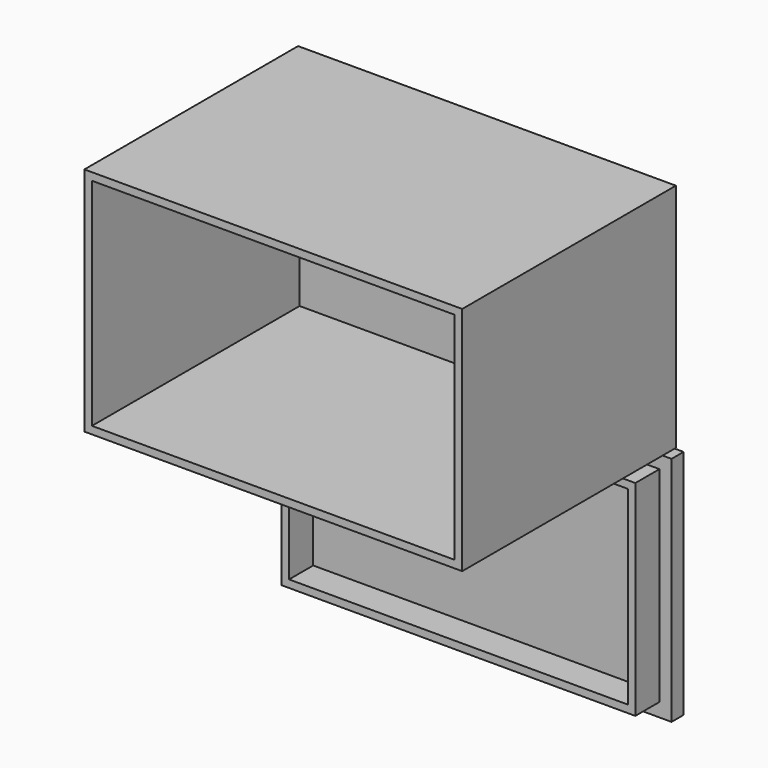
from build123d import *

# Parameters (mm, degrees)
F0_W        = 127.1928735077
F0_H        = 77.7173149399
F1_DEPTH    = 89.916
F2_T        = -2.54
F3_W        = 127.5507546961
F3_H        = 77.9658099636
F4_DEPTH    = 2.54
F5_W        = 119.1201396286
F5_H        = 69.0140379593
F6_DEPTH    = 10.16
F9_T        = 2.54
F9_T3_DEPTH = 124.2001396286
F9_T5_DEPTH = 74.0940379593
F8_W        = 127.5507546961
F8_H        = 77.9658099636
F8_W_2      = 46.9547603279
F8_H_2      = 47.2698919475
F8_W_3      = 21.6541066766
F8_H_3      = 15.249369666
F10_DEPTH   = 2.54


# Not quite as in the source:
# - a shell that OpenCascade refuses in one call is made with other operations: the cavity is built on its own and cut out


with BuildPart() as f1:
    # F0 (on Front) → F1 (new body)
    with BuildSketch(Plane.XZ):
        with Locations((-83.7561842054, 32.0948308799)):
            Rectangle(F0_W, F0_H)
    extrude(amount=F1_DEPTH)

    # F2
    f2_openings = [f1.faces().sort_by_distance(p)[0] for p in [
        (-83.756184, -89.916, 32.094831),
    ]]
    offset(amount=F2_T, openings=f2_openings)


with BuildPart() as f4:
    # F3 (on Front) → F4 (new body)
    with BuildSketch(Plane.XZ):
        with Locations((-83.3670627326, -47.7856700309)):
            Rectangle(F3_W, F3_H)
    extrude(amount=F4_DEPTH)

    # F5 (on face) → F6 (join)
    with BuildSketch(Plane.XZ.offset(2.54)):
        with Locations((-83.2092221826, -47.6696216501)):
            Rectangle(F5_W, F5_H)
    extrude(amount=F6_DEPTH)

    # F9: shell of thickness 2.54, made by hand


with BuildPart() as f9_core1:
    # F9_t2: copy of F4
    add(f4.part)

    # the walls: a layer under each face that stays
    f9_faces = [f9_core1.faces().sort_by_distance(p)[0] for p in [
        (-83.3670627326, -1.27, -8.802765049),
        (-19.5916853845, -1.27, -47.7856700309),
        (-147.1424400806, -1.27, -47.7856700309),
        (-83.3670627326, 0, -47.7856700309),
        (-142.8907482574, -2.54, -84.1697146806),
        (-83.3670627326, -1.27, -86.7685750127),
        (-83.2092221826, -7.62, -13.1626026705),
        (-142.769291997, -7.62, -47.6696216501),
        (-83.2092221826, -7.62, -82.1766406298),
        (-23.6491523683, -7.62, -47.6696216501),
    ]]
    thicken(f9_faces, amount=-F9_T, mode=Mode.SUBTRACT)

    # F9_s4 → F9_t3 (cut)
    with BuildSketch(Plane.YZ.offset(-145.309291997)):
        Polygon((-2.5654, -13.1372026705), (0, -13.1626026705), (0, -15.7026026705), (-2.54, -15.7026026705), align=None)
        Polygon((-2.5654, -82.2020406298), (0, -82.1766406298), (0, -79.6366406298), (-2.54, -79.6366406298), align=None)
    extrude(amount=F9_T3_DEPTH, mode=Mode.SUBTRACT)

    # F9_s6 → F9_t5 (cut)
    with BuildSketch(Plane.XY.offset(-84.7166406298)):
        Polygon((-142.794691997, -2.5654), (-142.769291997, 0), (-140.229291997, 0), (-140.229291997, -2.54), align=None)
        Polygon((-23.6237523683, -2.5654), (-23.6491523683, 0), (-26.1891523683, 0), (-26.1891523683, -2.54), align=None)
    extrude(amount=F9_T5_DEPTH, mode=Mode.SUBTRACT)


with BuildPart() as f4_1:
    add(f4.part)

    # what is left inside the walls is the cavity
    f9_cavity = [f9_core1.part.solids().sort_by_distance(p)[0] for p in [
        (-83.209222, -2.5654, -58.325295),
    ]]
    add(f9_cavity, mode=Mode.SUBTRACT)

    # F8 (on face) → F10 (join)
    with BuildSketch(Plane(origin=(0, 0, 0), x_dir=(-1, 0, 0), z_dir=(0, 1, 0))):
        with Locations((83.3670627326, -47.7856700309)):
            Rectangle(F8_W, F8_H)
        with Locations((54.326700978, -49.0877199918)):
            Rectangle(F8_W_2, F8_H_2, mode=Mode.SUBTRACT)
        with Locations((107.682403177, -33.5264848545)):
            Rectangle(F8_W_3, F8_H_3, mode=Mode.SUBTRACT)
    extrude(amount=F10_DEPTH)


solid = Compound([f1.part, f4_1.part])
